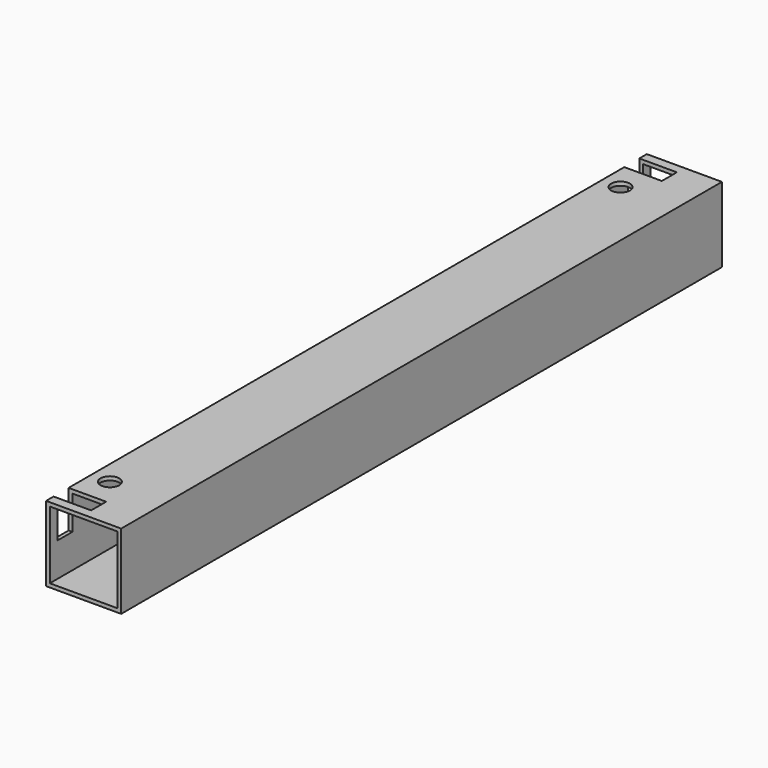
from build123d import *

# Parameters (mm, degrees)
F0_W     = 40
F0_H     = 40
F0_W_2   = 36
F0_H_2   = 36
F1_DEPTH = 200
F2_W     = 10
F2_H     = 30
F3_DEPTH = 20.001
F4_R     = 5
F5_DEPTH = 20.001


# Not quite as in the source:
# - a pattern or mirror of a feature is missing from the dataset's text; its kind, count and spacing are read off the source's solid


with BuildPart() as f1:
    # F0 (on Front) → F1 (new body, symmetric)
    with BuildSketch(Plane.XZ):
        Rectangle(F0_W, F0_H)
        Rectangle(F0_W_2, F0_H_2, mode=Mode.SUBTRACT)
    extrude(amount=F1_DEPTH, both=True)

    # F2 (on Right) → F3 (cut, through all)
    with BuildSketch(Plane.YZ):
        with Locations((-190, 15)):
            Rectangle(F2_W, F2_H)
    f3 = extrude(amount=-F3_DEPTH, mode=Mode.SUBTRACT)

    # F3_copies: F3 across plane
    add(f3.mirror(Plane.ZX), mode=Mode.SUBTRACT)

    # F4 (on Top) → F5 (cut, through all)
    with BuildSketch(Plane.XY):
        with Locations((-10, 170)):
            Circle(F4_R)
    f5 = extrude(amount=F5_DEPTH, mode=Mode.SUBTRACT)

    # F5_copies: F5 across plane
    add(f5.mirror(Plane(origin=(0, 0, 0), x_dir=(0, 0, -1), z_dir=(0, -1, 0))), mode=Mode.SUBTRACT)


solid = f1.part
